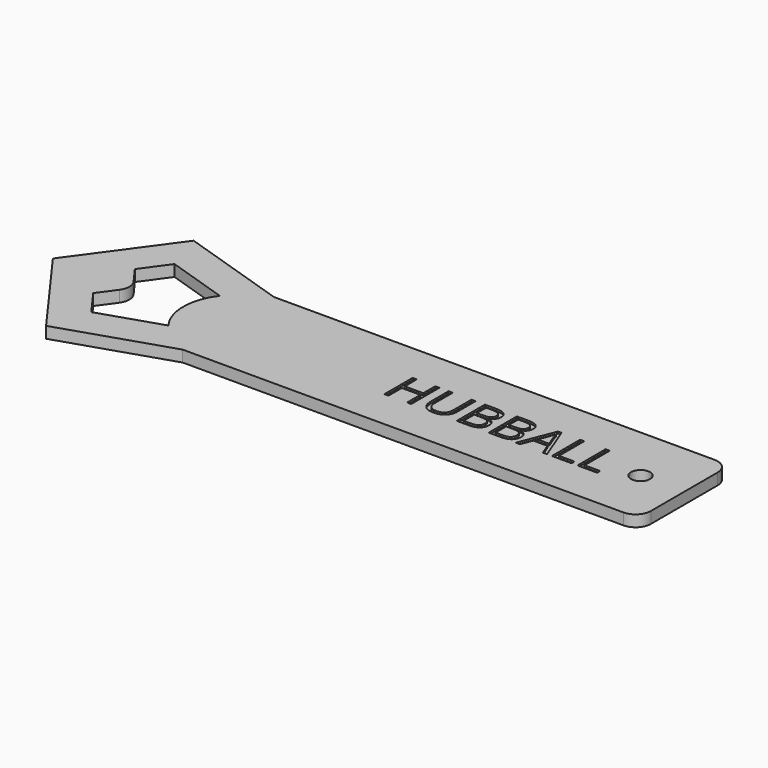
from build123d import *

# Parameters (mm, degrees)
F0_R         = 2.5
F1_DEPTH     = 3
F2_R         = 4
F3_TEXT_SIZE = 12.9819065074
F4_DEPTH     = 0.5


# Not quite as in the source:
# - Text() gives the source's letters only with a copy of the font that has no kerning and outlines rounded to 1/6400 em; it was checked with that copy


with BuildPart() as f1:
    # F0 (on Top) → F1 (new body)
    with BuildSketch(Plane.XY):
        Polygon((-7.8859666818, -24.2705098312), (20.6457288071, -15), (140.6457288071, -15), (140.6457288071, -3.7762515713), (140.6457288071, 0), (140.6457288071, 15), (20.6457288071, 15), (-7.8859666818, 24.2705098312), (-25.5195242506, 0), align=None)
        with BuildLine():
            ThreePointArc((11.6457288071, 8.461117248), (8.8002551347, 0), (11.6457288071, -8.461117248))
            Line((11.6457288071, -8.461117248), (-4.4482725805, -13.69037529))
            Line((-4.4482725805, -13.69037529), (-9.4215925168, -6.845187645))
            Line((-9.4215925168, -6.845187645), (-4.4482725805, 0))
            Line((-4.4482725805, 0), (-9.4215925168, 6.845187645))
            Line((-9.4215925168, 6.845187645), (-4.4482725805, 13.69037529))
            Line((-4.4482725805, 13.69037529), (11.6457288071, 8.461117248))
        make_face(mode=Mode.SUBTRACT)
        with Locations((129.1457288071, 0)):
            Circle(F0_R, mode=Mode.SUBTRACT)
    extrude(amount=F1_DEPTH)

    # F2
    f2_edges = [f1.edges().sort_by_distance(p)[0] for p in [
        (140.645729, -15, 1.5),
        (140.645729, 15, 1.5),
        (-4.448273, 0, 1.5),
    ]]
    fillet(f2_edges, radius=F2_R)

    # F3 (on face) → F4 (cut)
    with BuildSketch(Plane.XY.offset(3)):
        with Locations((64.1317665577, -4.5722937211)):
            Text('HUBBALL', F3_TEXT_SIZE, font='Open Sans', text_align=(TextAlign.LEFT, TextAlign.BOTTOM))
    extrude(amount=-F4_DEPTH, mode=Mode.SUBTRACT)


solid = f1.part
